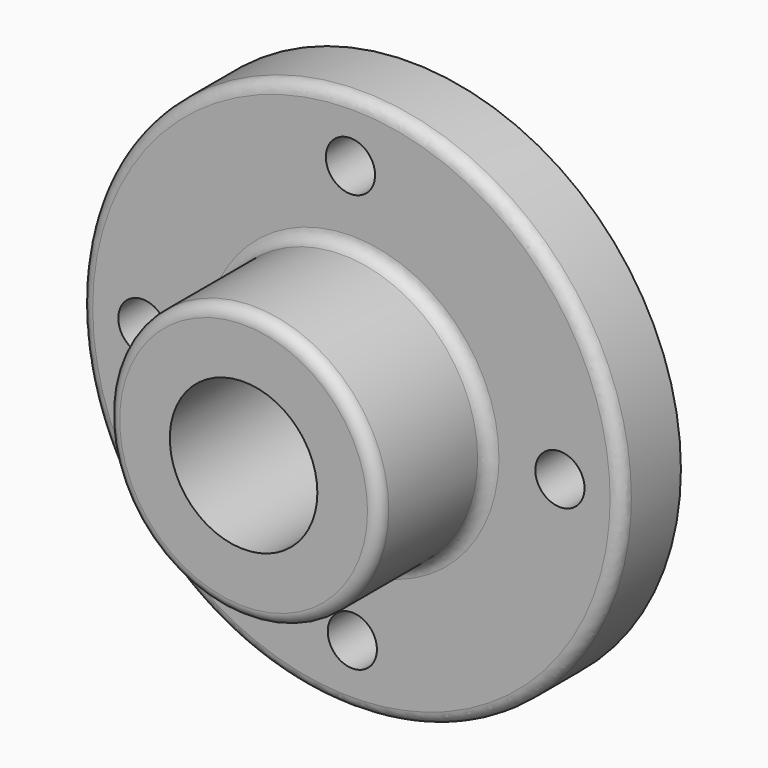
from build123d import *

# Parameters (mm, degrees)
F2_R            = 3.048
F3_R            = 6.35
F4_DEPTH        = 53.849
F4_COPIES_COUNT = 4


# Not quite as in the source:
# - a pattern or mirror of a feature is missing from the dataset's text; its kind, count and spacing are read off the source's solid


with BuildPart() as f1:
    # F0 (on Top) → F1 (revolve)
    with BuildSketch(Plane.XY):
        Polygon((50.8, 0), (0, 0), (0, -53.848), (15.9979741, -53.848), (15.9979741, -19.0510369452), (50.8, -19.05), align=None)
    revolve(axis=Axis((-19.05, -27.312900871, 0), (0, -1, 0)))

    # F2
    f2_edges = [f1.edges().sort_by_distance(p)[0] for p in [
        (-88.9, -19.05, 0),
        (-54.097974, -19.051037, 0),
        (-54.097974, -53.848, 0),
    ]]
    fillet(f2_edges, radius=F2_R)

    # F3 (on Front) → F4 (cut, through all)
    with BuildSketch(Plane.XZ):
        with Locations((-19.2909650505, 53.848)):
            Circle(F3_R)
    f4 = extrude(amount=F4_DEPTH, mode=Mode.SUBTRACT)

    # F4_copies: F4 ×4 about axis
    f4_copies_axis = Axis((-19.05, 0, 0), (0, 1, 0))
    for i in range(1, F4_COPIES_COUNT):
        add(f4.rotate(f4_copies_axis, i * 360 / F4_COPIES_COUNT), mode=Mode.SUBTRACT)


solid = f1.part
